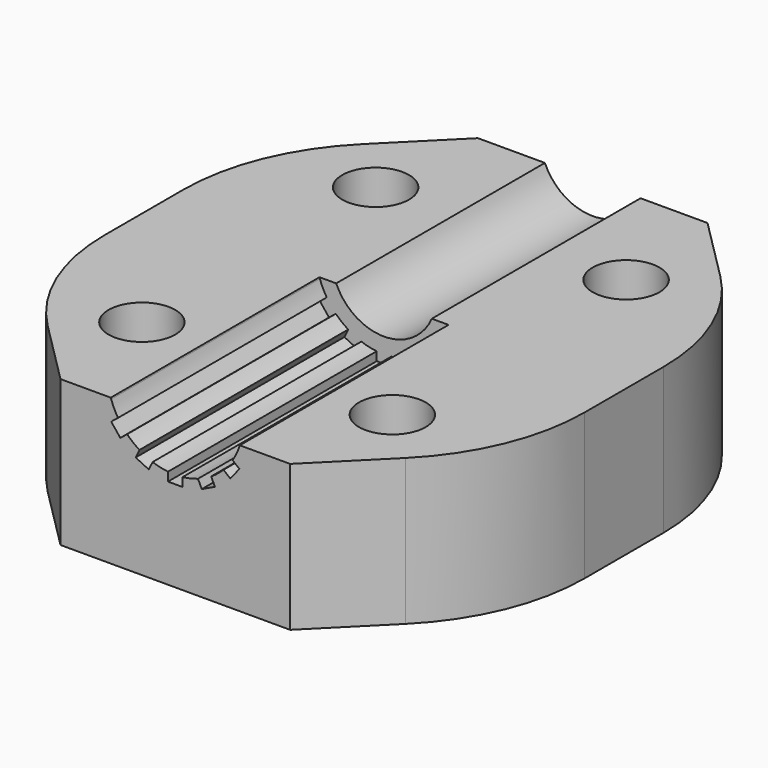
from build123d import *

# Parameters (mm, degrees)
F0_W      = 23
F0_H      = 25
F1_DEPTH  = 7
F3_DEPTH  = 25.001
F4_DEPTH  = 12.5
F5_SIZE   = 6
F6_R      = 10
F7_R      = 1.6
F8_DEPTH  = 25
F10_DEPTH = 2.5


with BuildPart() as f1:
    # F0 (on Top) → F1 (new body)
    with BuildSketch(Plane.XY):
        Rectangle(F0_W, F0_H)
    extrude(amount=F1_DEPTH)

    # F2 (on face) → F3 (cut, through all)
    with BuildSketch(Plane.XZ.offset(12.5)):
        with BuildLine():
            Line((0, 7), (-2.2912878475, 7))
            ThreePointArc((-2.2912878475, 7), (0, 5.5), (2.2912878475, 7))
            Line((2.2912878475, 7), (0, 7))
        make_face()
    extrude(amount=-F3_DEPTH, mode=Mode.SUBTRACT)

    # F2 (on face) → F4 (cut)
    with BuildSketch(Plane.XZ.offset(12.5)):
        with BuildLine():
            ThreePointArc((2.2912878475, 7), (0, 5.5), (-2.2912878475, 7))
            Line((-2.2912878475, 7), (-2.8084005449, 7))
            Line((-2.8084005449, 7), (-3.0722061624, 6.9397880893))
            ThreePointArc((-3.0722061624, 6.9397880893), (-2.9281488207, 6.5898778479), (-2.7443962613, 6.2590838157))
            Line((-2.7443962613, 6.2590838157), (-2.4464411557, 6.4966950836))
            Line((-2.4464411557, 6.4966950836), (-2.0099982944, 5.9494130458))
            Line((-2.0099982944, 5.9494130458), (-2.3079534, 5.711801778))
            ThreePointArc((-2.3079534, 5.711801778), (-2.026341856, 5.459047682), (-1.7172603691, 5.2407398048))
            Line((-1.7172603691, 5.2407398048), (-1.5519077603, 5.5840980352))
            Line((-1.5519077603, 5.5840980352), (-0.9212295527, 5.2803794178))
            Line((-0.9212295527, 5.2803794178), (-1.0865821616, 4.9370211875))
            ThreePointArc((-1.0865821616, 4.9370211875), (-0.7231930354, 4.8314842854), (-0.35, 4.7689011157))
            Line((-0.35, 4.7689011157), (-0.35, 5.15))
            Line((-0.35, 5.15), (0.35, 5.15))
            Line((0.35, 5.15), (0.35, 4.7689011157))
            ThreePointArc((0.35, 4.7689011157), (0.7231930354, 4.8314842854), (1.0865821616, 4.9370211875))
            Line((1.0865821616, 4.9370211875), (0.9212295527, 5.2803794178))
            Line((0.9212295527, 5.2803794178), (1.5519077603, 5.5840980352))
            Line((1.5519077603, 5.5840980352), (1.7172603691, 5.2407398048))
            ThreePointArc((1.7172603691, 5.2407398048), (2.026341856, 5.459047682), (2.3079534, 5.711801778))
            Line((2.3079534, 5.711801778), (2.0099982944, 5.9494130458))
            Line((2.0099982944, 5.9494130458), (2.4464411557, 6.4966950836))
            Line((2.4464411557, 6.4966950836), (2.7443962613, 6.2590838157))
            ThreePointArc((2.7443962613, 6.2590838157), (2.9281488207, 6.5898778479), (3.0722061624, 6.9397880893))
            Line((3.0722061624, 6.9397880893), (2.8084005449, 7))
            Line((2.8084005449, 7), (2.2912878475, 7))
        make_face()
        with BuildLine():
            Line((3.0719063417, 5.9979032421), (2.7443962613, 6.2590838157))
            ThreePointArc((2.7443962613, 6.2590838157), (2.540952318, 5.973658144), (2.3079534, 5.711801778))
            Line((2.3079534, 5.711801778), (2.6354634804, 5.4506212044))
            Line((2.6354634804, 5.4506212044), (3.0719063417, 5.9979032421))
        make_face()
        with BuildLine():
            ThreePointArc((2.3079534, 5.711801778), (2.540952318, 5.973658144), (2.7443962613, 6.2590838157))
            Line((2.7443962613, 6.2590838157), (2.4464411557, 6.4966950836))
            Line((2.4464411557, 6.4966950836), (2.0099982944, 5.9494130458))
            Line((2.0099982944, 5.9494130458), (2.3079534, 5.711801778))
        make_face()
        with BuildLine():
            Line((1.8990147515, 4.8633229408), (1.7172603691, 5.2407398048))
            ThreePointArc((1.7172603691, 5.2407398048), (1.4101221521, 5.0718511793), (1.0865821616, 4.9370211875))
            Line((1.0865821616, 4.9370211875), (1.268336544, 4.5596043235))
            Line((1.268336544, 4.5596043235), (1.8990147515, 4.8633229408))
        make_face()
        with BuildLine():
            ThreePointArc((1.0865821616, 4.9370211875), (1.4101221521, 5.0718511793), (1.7172603691, 5.2407398048))
            Line((1.7172603691, 5.2407398048), (1.5519077603, 5.5840980352))
            Line((1.5519077603, 5.5840980352), (0.9212295527, 5.2803794178))
            Line((0.9212295527, 5.2803794178), (1.0865821616, 4.9370211875))
        make_face()
        with BuildLine():
            ThreePointArc((0.35, 4.7689011157), (0, 4.75), (-0.35, 4.7689011157))
            Line((-0.35, 4.7689011157), (-0.35, 4.35))
            Line((-0.35, 4.35), (0.35, 4.35))
            Line((0.35, 4.35), (0.35, 4.7689011157))
        make_face()
        with BuildLine():
            Line((-0.35, 5.15), (-0.35, 4.7689011157))
            ThreePointArc((-0.35, 4.7689011157), (0, 4.75), (0.35, 4.7689011157))
            Line((0.35, 4.7689011157), (0.35, 5.15))
            Line((0.35, 5.15), (-0.35, 5.15))
        make_face()
        with BuildLine():
            ThreePointArc((-1.0865821616, 4.9370211875), (-1.4101221521, 5.0718511793), (-1.7172603691, 5.2407398048))
            Line((-1.7172603691, 5.2407398048), (-1.8990147515, 4.8633229408))
            Line((-1.8990147515, 4.8633229408), (-1.268336544, 4.5596043235))
            Line((-1.268336544, 4.5596043235), (-1.0865821616, 4.9370211875))
        make_face()
        with BuildLine():
            Line((-1.5519077603, 5.5840980352), (-1.7172603691, 5.2407398048))
            ThreePointArc((-1.7172603691, 5.2407398048), (-1.4101221521, 5.0718511793), (-1.0865821616, 4.9370211875))
            Line((-1.0865821616, 4.9370211875), (-0.9212295527, 5.2803794178))
            Line((-0.9212295527, 5.2803794178), (-1.5519077603, 5.5840980352))
        make_face()
        with BuildLine():
            ThreePointArc((-2.3079534, 5.711801778), (-2.540952318, 5.973658144), (-2.7443962613, 6.2590838157))
            Line((-2.7443962613, 6.2590838157), (-3.0719063417, 5.9979032421))
            Line((-3.0719063417, 5.9979032421), (-2.6354634804, 5.4506212044))
            Line((-2.6354634804, 5.4506212044), (-2.3079534, 5.711801778))
        make_face()
        with BuildLine():
            Line((-2.4464411557, 6.4966950836), (-2.7443962613, 6.2590838157))
            ThreePointArc((-2.7443962613, 6.2590838157), (-2.540952318, 5.973658144), (-2.3079534, 5.711801778))
            Line((-2.3079534, 5.711801778), (-2.0099982944, 5.9494130458))
            Line((-2.0099982944, 5.9494130458), (-2.4464411557, 6.4966950836))
        make_face()
        with BuildLine():
            Line((3.0923292192, 7), (2.8084005449, 7))
            Line((2.8084005449, 7), (3.0722061624, 6.9397880893))
            ThreePointArc((3.0722061624, 6.9397880893), (3.0824147168, 6.969844908), (3.0923292192, 7))
        make_face()
        with BuildLine():
            Line((-3.0722061624, 6.9397880893), (-2.8084005449, 7))
            Line((-2.8084005449, 7), (-3.0923292192, 7))
            ThreePointArc((-3.0923292192, 7), (-3.0824147168, 6.969844908), (-3.0722061624, 6.9397880893))
        make_face()
    extrude(amount=-F4_DEPTH, mode=Mode.SUBTRACT)

    # F5
    f5_edges = [f1.edges().sort_by_distance(p)[0] for p in [
        (11.5, -12.5, 3.5),
        (-11.5, -12.5, 3.5),
        (11.5, 12.5, 3.5),
        (-11.5, 12.5, 3.5),
    ]]
    chamfer(f5_edges, length=F5_SIZE)

    # F6
    f6_edges = [f1.edges().sort_by_distance(p)[0] for p in [
        (11.5, 6.5, 3.5),
        (11.5, -6.5, 3.5),
        (-11.5, 6.5, 3.5),
        (-11.5, -6.5, 3.5),
    ]]
    fillet(f6_edges, radius=F6_R)

    # F7 (on face) → F8 (cut)
    with BuildSketch(Plane.XY.offset(7)):
        with Locations((6, -7)):
            Circle(F7_R)
        with Locations((-6, -7)):
            Circle(F7_R)
        with Locations((-6, 7)):
            Circle(F7_R)
        with Locations((6, 7)):
            Circle(F7_R)
    extrude(amount=-F8_DEPTH, mode=Mode.SUBTRACT)

    # F9 (on face) → F10 (cut)
    with BuildSketch(Plane(origin=(0, 0, 0), x_dir=(1, 0, 0), z_dir=(0, 0, -1))):
        Polygon((-4.3545517328, 4.15), (-2.7091034656, 7), (-4.3545517328, 9.85), (-7.6454482672, 9.85), (-9.2908965344, 7), (-7.6454482672, 4.15), align=None)
        Polygon((-9.2908965344, -7), (-7.6454482672, -9.85), (-4.3545517328, -9.85), (-2.7091034656, -7), (-4.3545517328, -4.15), (-7.6454482672, -4.15), align=None)
        Polygon((2.7091034656, 7), (4.3545517328, 4.15), (7.6454482672, 4.15), (9.2908965344, 7), (7.6454482672, 9.85), (4.3545517328, 9.85), align=None)
        Polygon((2.7091034656, -7), (4.3545517328, -9.85), (7.6454482672, -9.85), (9.2908965344, -7), (7.6454482672, -4.15), (4.3545517328, -4.15), align=None)
    extrude(amount=-F10_DEPTH, mode=Mode.SUBTRACT)


solid = f1.part
